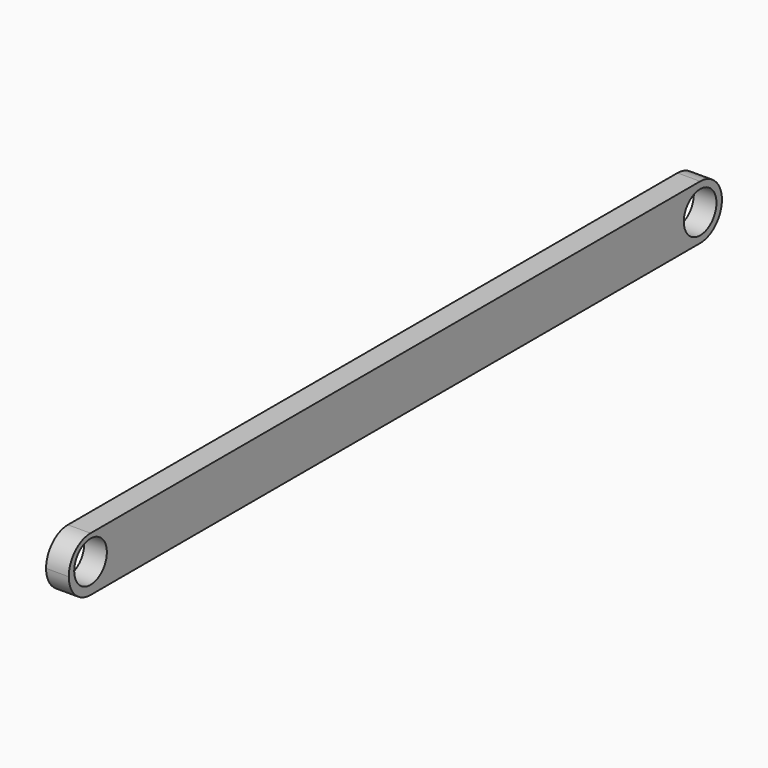
from build123d import *

# Parameters (mm, degrees)
F0_W     = 2.5
F0_H     = 6
F1_DEPTH = 90
F2_R     = 2.25
F3_DEPTH = 25
F4_R     = 2.99999
F5_R     = 2.25
F6_DEPTH = 25
F7_R     = 2.99999


# Not quite as in the source:
# - a fillet or chamfer is up to 0.001 mm smaller than in the source, because OpenCascade refuses the exact size


with BuildPart() as f1:
    # F0 (on Front) → F1 (new body)
    with BuildSketch(Plane.XZ):
        Rectangle(F0_W, F0_H)
    extrude(amount=F1_DEPTH)

    # F2 (on face) → F3 (cut)
    with BuildSketch(Plane(origin=(-1.25, 0, 0), x_dir=(0, -1, 0), z_dir=(-1, 0, 0))):
        with Locations((3, 0)):
            Circle(F2_R)
    extrude(amount=-F3_DEPTH, mode=Mode.SUBTRACT)

    # F4 (radius 3 in the source; OpenCascade refuses exactly that, so slightly less here)
    f4_edges = [f1.edges().sort_by_distance(p)[0] for p in [
        (0, 0, 3),
        (0, 0, -3),
    ]]
    fillet(f4_edges, radius=F4_R)

    # F5 (on face) → F6 (cut)
    with BuildSketch(Plane(origin=(-1.25, 0, 0), x_dir=(0, -1, 0), z_dir=(-1, 0, 0))):
        with Locations((87, 0.2363782405)):
            Circle(F5_R)
    extrude(amount=-F6_DEPTH, mode=Mode.SUBTRACT)

    # F7 (radius 3 in the source; OpenCascade refuses exactly that, so slightly less here)
    f7_edges = [f1.edges().sort_by_distance(p)[0] for p in [
        (0, -90, 3),
        (0, -90, -3),
    ]]
    fillet(f7_edges, radius=F7_R)


solid = f1.part
